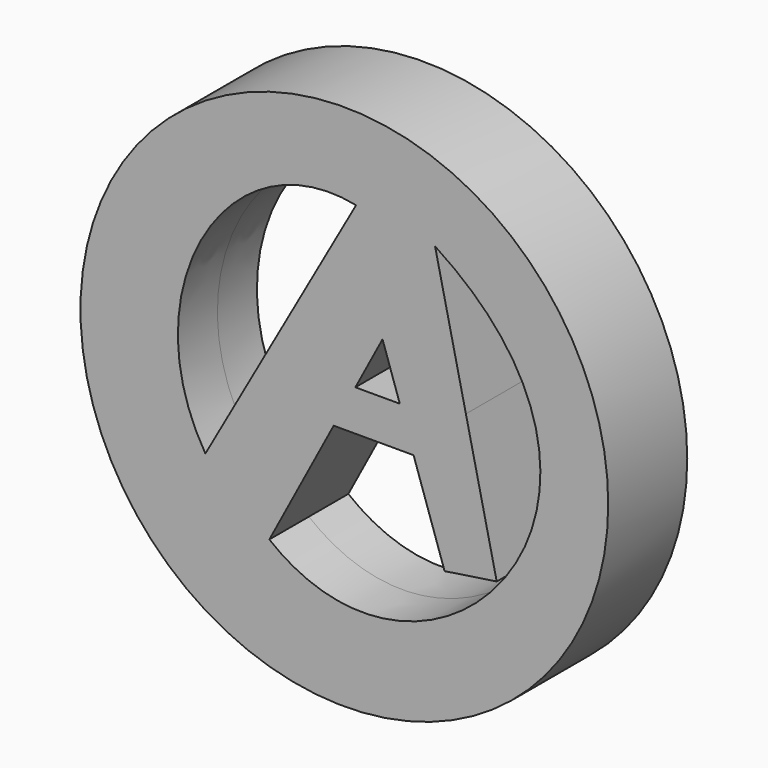
from build123d import *

# Parameters (mm, degrees)
F0_R     = 67.8507584939
F1_DEPTH = 12.7
F2_DEPTH = 12.7
F3_DEPTH = 12.7


# Not quite as in the source:
# - a feature of the source that left no trace in its solid (it failed there, or was rolled back) is left out


with BuildPart() as f1:
    # F0 (on Front) → F1 (new body, symmetric)
    with BuildSketch(Plane.XZ):
        with Locations((6.3937897791, -10.4070244153)):
            Circle(F0_R)
        with BuildLine():
            Line((16.2108500706, 8.0759122229), (29.7189755197, 33.5081515453))
            add(Edge.make_bspline(
                [(29.7189755197, 33.5081515453), (93.8960388303, -7.9348757863), (29.3413570435, -80.48370842), (-12.8972016539, -46.7268759549)],
                knots=[0, 0, 0, 0, 90.8504165915, 90.8504165915, 90.8504165915, 90.8504165915], degree=3))
            Line((-12.8972016539, -46.7268759549), (3.6481818786, -15.5762803179))
            Line((3.6481818786, -15.5762803179), (9.2231951319, -5.08))
            Line((9.2231951319, -5.08), (16.2108500706, 8.0759122229))
        make_face(mode=Mode.SUBTRACT)
        with BuildLine():
            Line((9.4068207245, 36.2007932827), (-29.3430900942, -32.6330686977))
            add(Edge.make_bspline(
                [(-29.3430900942, -32.6330686977), (-49.592975527, 0), (-23.1433883309, 42.9805777967), (9.4068207245, 36.2007932827)],
                knots=[0, 0, 0, 0, 78.9914941218, 78.9914941218, 78.9914941218, 78.9914941218], degree=3))
        make_face(mode=Mode.SUBTRACT)
    extrude(amount=F1_DEPTH, both=True)

    # F0 (on Front) → F2 (join, symmetric)
    with BuildSketch(Plane.XZ):
        Polygon((37.6452035187, -1.8549078334), (29.7189755197, 33.5081515453), (16.2108500706, 8.0759122229), (20.6487422011, -5.08), (24.1894590312, -15.5762803179), (32.1680679917, -39.2284728587), (45.5714315176, -37.2179672122), align=None)
    extrude(amount=F2_DEPTH, both=True)

    # F0 (on Front) → F3 (join, symmetric)
    with BuildSketch(Plane.XZ):
        Polygon((20.6487422011, -5.08), (9.2231951319, -5.08), (3.6481818786, -15.5762803179), (24.1894590312, -15.5762803179), align=None)
    extrude(amount=F3_DEPTH, both=True)


solid = f1.part
